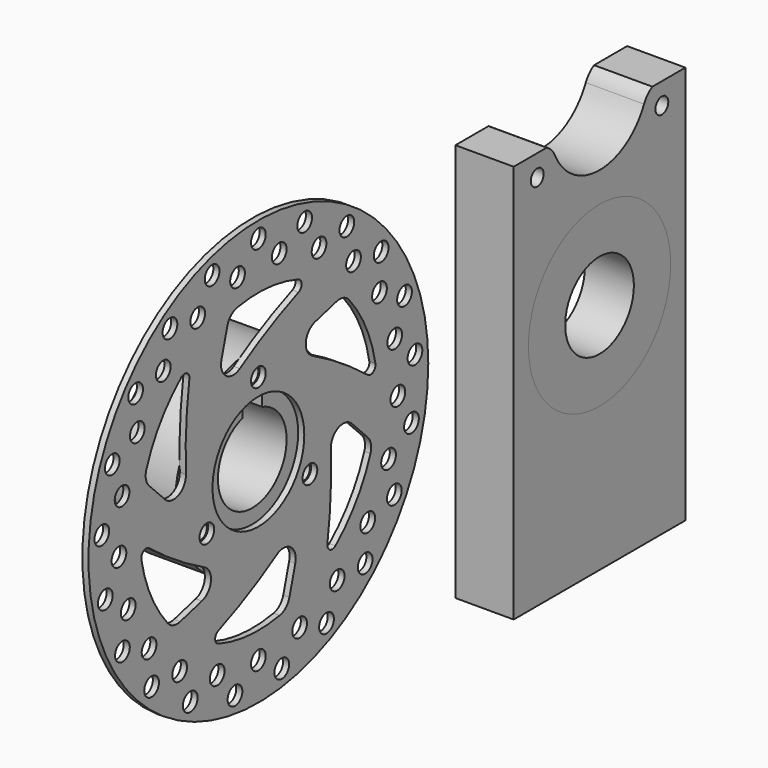
from build123d import *

# Parameters (mm, degrees)
F0_R             = 69.25
F0_R_2           = 18.7
F1_DEPTH         = 2
F3_D             = 6
F5_D             = 6
F7_D             = 6
F9_DEPTH         = 2.001
F9_COPIES_COUNT  = 6
F10_R            = 5
F11_R            = 2
F12_R            = 31.5
F12_R_2          = 14
F13_DEPTH        = 20
F15_DEPTH        = 22.0010001
F17_D            = 5
F17_COPIES_COUNT = 3
F18_R            = 29
F18_R_2          = 14
F19_DEPTH        = 16
F20_W            = 70
F20_H            = 130
F20_R            = 25
F21_DEPTH        = 3
F21_DEPTH_BACK   = 16
F22_R            = 29
F23_DEPTH        = 16
F25_D            = 5.25
F27_DEPTH        = 36.001
F29_D            = 5
F29_DEPTH        = 30
F29_TIP          = 1.5021515476


# Not quite as in the source:
# - a pattern or mirror of a feature is missing from the dataset's text; its kind, count and spacing are read off the source's solid


with BuildPart() as f1:
    # F0 (on Right) → F1 (new body)
    with BuildSketch(Plane.YZ):
        Circle(F0_R)
        Circle(F0_R_2, mode=Mode.SUBTRACT)
    extrude(amount=F1_DEPTH)

    # F3 (through all)
    with Locations(Plane.YZ.offset(2)):
        with Locations((0, 24.25), (-21.0011160418, -12.125), (21.0011160418, -12.125)):
            Hole(F3_D / 2)

    # F5 (through all)
    with Locations(Plane.YZ.offset(2)):
        with Locations((0, 64), (18.8643311623, 61.1566595703), (36.0524837161, 52.8792815562), (50.037214878, 39.903347319), (59.5759199132, 23.3818255594), (63.8210430196, 4.7827259895), (62.3953863796, -14.2413397732), (55.4256258422, -32), (43.5310552173, -46.9153197971), (27.7685593035, -57.6620075458), (9.5387050353, -63.2851728784), (-9.5387050353, -63.2851728784), (-27.7685593035, -57.6620075458), (-43.5310552173, -46.9153197971), (-55.4256258422, -32), (-62.3953863796, -14.2413397732), (-63.8210430196, 4.7827259895), (-59.5759199132, 23.3818255594), (-50.037214878, 39.903347319), (-36.0524837161, 52.8792815562), (-18.8643311623, 61.1566595703)):
            Hole(F5_D / 2)

    # F7 (through all)
    with Locations(Plane.YZ.offset(2)):
        with Locations((0, -57), (-16.8010449414, -54.4676499298), (-32.1092433096, -47.095610136), (-44.5643945007, -35.5389187059), (-53.0598036727, -20.8244383889), (-56.8406164393, -4.2596153344), (-55.5708909944, 12.6836932355), (-49.3634480157, 28.5), (-38.7698460529, 41.7839566943), (-24.7313731297, 51.3552254704), (-8.495409172, 56.3633570948), (8.495409172, 56.3633570948), (24.7313731297, 51.3552254704), (38.7698460529, 41.7839566943), (49.3634480157, 28.5), (55.5708909944, 12.6836932355), (56.8406164393, -4.2596153344), (53.0598036727, -20.8244383889), (44.5643945007, -35.5389187059), (32.1092433096, -47.095610136), (16.8010449414, -54.4676499298)):
            Hole(F7_D / 2)

    # F8 (on face) → F9 (cut, through all)
    with BuildSketch(Plane.YZ.offset(2)):
        with BuildLine():
            ThreePointArc((-18.7117130734, 21.9572819575), (0.3120725782, 34.3893720191), (21.044690473, 43.6963499951))
            ThreePointArc((21.044690473, 43.6963499951), (4.8954910444, 48.2522970172), (-11.8396757075, 47.0326703382))
            Line((-11.8396757075, 47.0326703382), (-18.7117130734, 21.9572819575))
        make_face()
    f9 = extrude(amount=-F9_DEPTH, mode=Mode.SUBTRACT)

    # F9_copies: F9 ×6 about axis
    f9_copies_axis = Axis((0, 0, 0), (1, 0, 0))
    for i in range(1, F9_COPIES_COUNT):
        add(f9.rotate(f9_copies_axis, i * 360 / F9_COPIES_COUNT), mode=Mode.SUBTRACT)

    # F10
    f10_edges = [f1.edges().sort_by_distance(p)[0] for p in [
        (1, -11.839676, 47.03267),
        (1, -18.711713, 21.957282),
        (1, 11.839676, -47.03267),
        (1, 18.711713, -21.957282),
        (1, -34.811649, -33.769795),
        (1, -9.659707, -27.18346),
        (1, 46.651325, -13.262875),
        (1, 28.371421, 5.226178),
        (1, -46.651325, 13.262875),
        (1, -28.371421, -5.226178),
        (1, 34.811649, 33.769795),
        (1, 9.659707, 27.18346),
    ]]
    fillet(f10_edges, radius=F10_R)

    # F11
    f11_edges = [f1.edges().sort_by_distance(p)[0] for p in [
        (1, 21.04469, 43.69635),
        (1, -21.04469, -43.69635),
        (1, -48.364494, -3.622938),
        (1, 27.319804, -40.073412),
        (1, -27.319804, 40.073412),
        (1, 48.364494, 3.622938),
    ]]
    fillet(f11_edges, radius=F11_R)


with BuildPart() as f13:
    # F12 (on face) → F13 (new body)
    with BuildSketch(Plane(origin=(0, 0, 0), x_dir=(0, -1, 0), z_dir=(-1, 0, 0))):
        Circle(F12_R)
        Circle(F12_R_2, mode=Mode.SUBTRACT)
    extrude(amount=F13_DEPTH)

    # F14 (on face) → F15 (cut, through all)
    with BuildSketch(Plane(origin=(-20, 0, 0), x_dir=(0, -1, 0), z_dir=(-1, 0, 0))):
        with BuildLine():
            Line((4, 17.8), (-4, 17.8))
            Line((-4, 17.8), (-4, 13.416407865))
            ThreePointArc((-4, 13.416407865), (0, 14), (4, 13.416407865))
            Line((4, 13.416407865), (4, 17.8))
        make_face()
    extrude(amount=-F15_DEPTH, mode=Mode.SUBTRACT)

    # F17 (through all)
    with Locations(Plane.YZ):
        with Locations((0, 24.25)):
            f17 = Hole(F17_D / 2)

    # F17_copies: F17 ×3 about axis
    f17_copies_axis = Axis((0, 0, 0), (1, 0, 0))
    for i in range(1, F17_COPIES_COUNT):
        add(f17.rotate(f17_copies_axis, i * 360 / F17_COPIES_COUNT), mode=Mode.SUBTRACT)


with BuildPart() as f19:
    # F18 (on Right) → F19 (new body)
    with BuildSketch(Plane.YZ):
        with Locations((121.5566498835, 0)):
            Circle(F18_R)
        with Locations((121.5566498835, 0)):
            Circle(F18_R_2, mode=Mode.SUBTRACT)
    extrude(amount=F19_DEPTH)


with BuildPart() as f21:
    # F20 (on face) → F21 (new body, two sides)
    with BuildSketch(Plane(origin=(0, 0, 0), x_dir=(0, -1, 0), z_dir=(-1, 0, 0))) as f21_sk:
        with Locations((-121.5566498835, -11)):
            Rectangle(F20_W, F20_H)
        with Locations((-121.5566498835, 0)):
            Circle(F20_R, mode=Mode.SUBTRACT)
    extrude(amount=F21_DEPTH)
    extrude(f21_sk.sketch, amount=-F21_DEPTH_BACK)

    # F22 (on face) → F23 (cut)
    with BuildSketch(Plane.YZ.offset(16)):
        with Locations((121.5566498835, 0)):
            Circle(F22_R)
    extrude(amount=-F23_DEPTH, mode=Mode.SUBTRACT)

    # F25 (through all)
    with Locations(Plane(origin=(-3, 0, 0), x_dir=(0, -1, 0), z_dir=(-1, 0, 0))):
        with Locations((-96.1566498835, 47), (-146.9566498835, 47)):
            Hole(F25_D / 2)

    # F26 (on face) → F27 (cut, through all)
    with BuildSketch(Plane.YZ.offset(16)):
        with BuildLine():
            ThreePointArc((100.0296332297, 54), (102.0107388866, 52.452489518), (103.4137927407, 50.3665824735))
            ThreePointArc((103.4137927407, 50.3665824735), (121.5566498835, 38.7830386573), (139.6995070264, 50.3665824735))
            ThreePointArc((139.6995070264, 50.3665824735), (141.1025608804, 52.452489518), (143.0836665373, 54))
            Line((143.0836665373, 54), (100.0296332297, 54))
        make_face()
    extrude(amount=-F27_DEPTH, mode=Mode.SUBTRACT)

    # F29
    with Locations(Plane(origin=(0, 0, -76), x_dir=(1, 0, 0), z_dir=(0, 0, -1))):
        with Locations((6.5, -112.1566498835), (6.5, -130.9566498835)):
            Hole(F29_D / 2, depth=F29_DEPTH)
            with Locations((0, 0, -(F29_DEPTH + F29_TIP / 2))):  # 118° drill point
                Cone(0, F29_D / 2, F29_TIP, mode=Mode.SUBTRACT)


solid = Compound([f1.part, f13.part, f19.part, f21.part])
